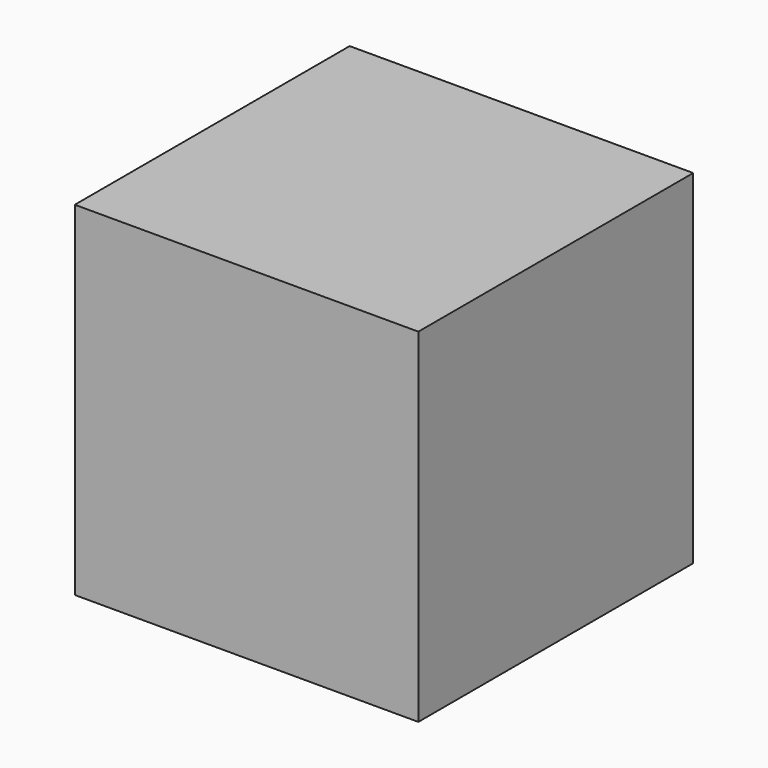
from build123d import *

# Parameters (mm, degrees)
F1_W     = 254
F1_H     = 254
F2_DEPTH = 254


# Not quite as in the source:
# - a variable given as a bare number and used for a length is read in inches; the dataset says mm whatever the document's units were


with BuildPart() as f2:
    # F1 (on Top) → F2 (new body)
    with BuildSketch(Plane.XY):
        with Locations((127, 127)):
            Rectangle(F1_W, F1_H)
    extrude(amount=F2_DEPTH)


solid = f2.part
